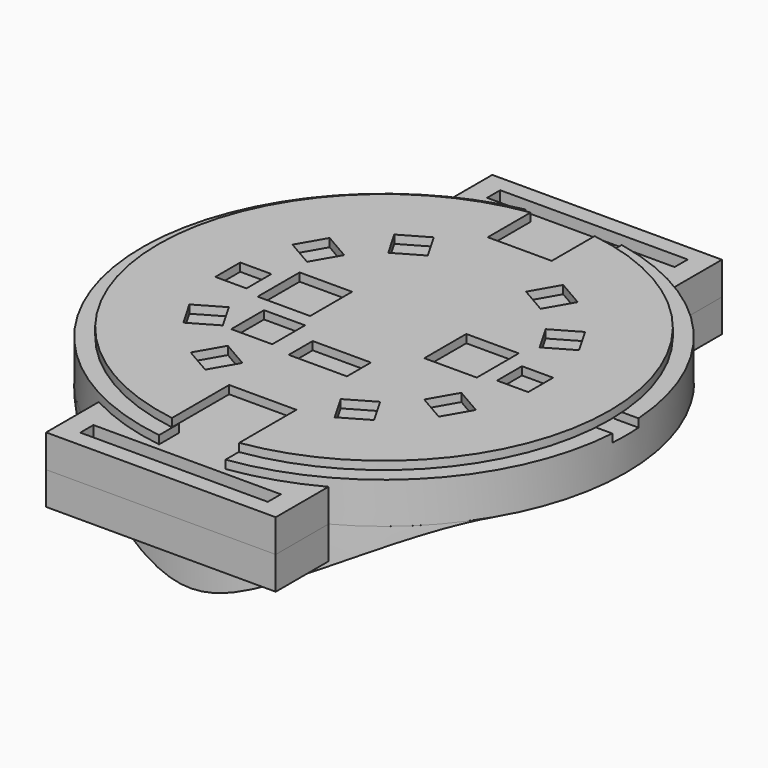
from build123d import *

# Parameters (mm, degrees)
F0_R      = 29.5
F0_R_2    = 26.5
F1_DEPTH  = 4
F3_DEPTH  = 1
F5_DEPTH  = 29.501
F7_DEPTH  = 29.501
F9_DEPTH  = 34
F10_W     = 22.86
F10_H     = 2
F11_DEPTH = 4.001
F13_DEPTH = 29.501
F14_R     = 27.5
F16_DEPTH = 1
F15_W     = 3.8
F15_H     = 3.8
F15_W_2   = 6.4
F15_H_2   = 6.4
F15_W_3   = 5
F15_H_3   = 5
F15_W_4   = 7.1
F15_H_4   = 3.65
F15_W_5   = 7.8
F15_H_5   = 8
F15_W_6   = 8.2
F15_H_6   = 10.85
F17_DEPTH = 25
F18_R     = 29.5
F19_DEPTH = 10
F22_DEPTH = 50
F18_W     = 22.86
F18_H     = 2
F23_DEPTH = 4
F24_DEPTH = 4


with BuildPart() as f1:
    # F0 (on Top) → F1 (new body)
    with BuildSketch(Plane.XY):
        Circle(F0_R)
        Circle(F0_R_2, mode=Mode.SUBTRACT)
        Circle(F0_R_2)
    extrude(amount=-F1_DEPTH)

    # F0 (on Top) → F3 (join)
    with BuildSketch(Plane.XY):
        Circle(F0_R)
        Circle(F0_R_2, mode=Mode.SUBTRACT)
    extrude(amount=F3_DEPTH)

    # F4 (on Front) → F5 (cut, through all)
    with BuildSketch(Plane.XZ):
        Polygon((-4.05, 0), (0, 0), (4.05, 0), (4.05, 3), (-4.05, 3), align=None)
    extrude(amount=F5_DEPTH, mode=Mode.SUBTRACT)

    # F6 (on Front) → F7 (cut, through all)
    with BuildSketch(Plane.XZ):
        Polygon((-5.85, 0), (0, 0), (5.85, 0), (5.85, 3), (-5.85, 3), align=None)
    extrude(amount=-F7_DEPTH, mode=Mode.SUBTRACT)

    # F8 (on Front) → F9 (join, symmetric)
    with BuildSketch(Plane.XZ):
        Polygon((14, 0), (0, 0), (-14, 0), (-14, -4), (14, -4), align=None)
    extrude(amount=F9_DEPTH, both=True)

    # F10 (on face) → F11 (cut, through all)
    with BuildSketch(Plane.XY):
        with Locations((0, 31)):
            Rectangle(F10_W, F10_H)
        with Locations((0, -31)):
            Rectangle(F10_W, F10_H)
    extrude(amount=-F11_DEPTH, mode=Mode.SUBTRACT)

    # F12 (on Right) → F13 (cut, through all)
    with BuildSketch(Plane.YZ):
        Polygon((-2, 0), (0, 0), (2, 0), (2, 3), (0, 3), (-2, 3), align=None)
    extrude(amount=F13_DEPTH, mode=Mode.SUBTRACT)


with BuildPart() as f16:
    # F14 (on face) → F16 (new body)
    with BuildSketch(Plane.XY.offset(1)):
        Circle(F14_R)
    extrude(amount=F16_DEPTH)

    # F15 (on face) → F17 (cut)
    with BuildSketch(Plane.XY.offset(1)):
        with Locations((-17.15, 0)):
            Rectangle(F15_W, F15_H)
        with Locations((-10.16, 0.64)):
            Rectangle(F15_W_2, F15_H_2)
        with Locations((-8.64, -6.86)):
            Rectangle(F15_W_3, F15_H_3)
        with Locations((0, -8.26)):
            Rectangle(F15_W_4, F15_H_4)
        with Locations((10.16, 0.64)):
            Rectangle(F15_W_2, F15_H_2)
        Polygon((-14.1413541181, -5.9753896004), (-17.4322506525, -7.8753896004), (-15.5322506525, -11.1662861348), (-12.2413541181, -9.2662861348), align=None)
        Polygon((-9.2435438204, -12.2413541181), (-11.1435438204, -15.5322506525), (-7.852647286, -17.4322506525), (-5.952647286, -14.1413541181), align=None)
        Polygon((6.0064561796, -14.1102875389), (7.9064561796, -17.4011840733), (11.197352714, -15.5011840733), (9.297352714, -12.2102875389), align=None)
        Polygon((12.2724206973, -9.2124772412), (15.5633172317, -11.1124772412), (17.4633172317, -7.8215807068), (14.1724206973, -5.9215807068), align=None)
        with Locations((17.15, 0.0621331584)):
            Rectangle(F15_W, F15_H)
        Polygon((14.1413541181, 6.0375227588), (17.4322506525, 7.9375227588), (15.5322506525, 11.2284192932), (12.2413541181, 9.3284192932), align=None)
        Polygon((9.2435438204, 12.3034872765), (11.1435438204, 15.5943838109), (7.852647286, 17.4943838109), (5.952647286, 14.2034872765), align=None)
        Polygon((-6.0064561796, 14.1724206973), (-7.9064561796, 17.4633172317), (-11.197352714, 15.5633172317), (-9.297352714, 12.2724206973), align=None)
        Polygon((-12.2724206973, 9.2746103996), (-15.5633172317, 11.1746103996), (-17.4633172317, 7.8837138652), (-14.1724206973, 5.9837138652), align=None)
        with Locations((0, 24.69)):
            Rectangle(F15_W_5, F15_H_5)
        with Locations((0, -23.9)):
            Rectangle(F15_W_6, F15_H_6)
    extrude(amount=F17_DEPTH, mode=Mode.SUBTRACT)


with BuildPart() as f19:
    # F18 (on face) → F19 (new body)
    with BuildSketch(Plane(origin=(0, 0, -4), x_dir=(1, 0, 0), z_dir=(0, 0, -1))):
        Circle(F18_R)
    extrude(amount=F19_DEPTH)

    # F21 (on Right) → F22 (cut, symmetric)
    with BuildSketch(Plane.YZ):
        with BuildLine():
            Line((-29.5, -14), (0, -14))
            Line((0, -14), (29.5, -14))
            ThreePointArc((29.5, -14), (23.8069574769, -6.7424116585), (15, -4))
            Line((15, -4), (0, -4))
            Line((0, -4), (-15, -4))
            ThreePointArc((-15, -4), (-23.8069574769, -6.7424116585), (-29.5, -14))
        make_face()
    extrude(amount=F22_DEPTH, both=True, mode=Mode.SUBTRACT)

    # F18 (on face) → F23 (join)
    with BuildSketch(Plane(origin=(0, 0, -4), x_dir=(1, 0, 0), z_dir=(0, 0, -1))):
        with BuildLine():
            Line((14, -34), (14, -25.9663243452))
            ThreePointArc((14, -25.9663243452), (0, -29.5), (-14, -25.9663243452))
            Line((-14, -25.9663243452), (-14, -34))
            Line((-14, -34), (14, -34))
        make_face()
        with Locations((0, -31)):
            Rectangle(F18_W, F18_H, mode=Mode.SUBTRACT)
    extrude(amount=F23_DEPTH)

    # F18 (on face) → F24 (join)
    with BuildSketch(Plane(origin=(0, 0, -4), x_dir=(1, 0, 0), z_dir=(0, 0, -1))):
        with BuildLine():
            ThreePointArc((-14, 25.9663243452), (0, 29.5), (14, 25.9663243452))
            Line((14, 25.9663243452), (14, 34))
            Line((14, 34), (-14, 34))
            Line((-14, 34), (-14, 25.9663243452))
        make_face()
        with Locations((0, 31)):
            Rectangle(F18_W, F18_H, mode=Mode.SUBTRACT)
    extrude(amount=F24_DEPTH)


solid = Compound([f1.part, f16.part, f19.part])
